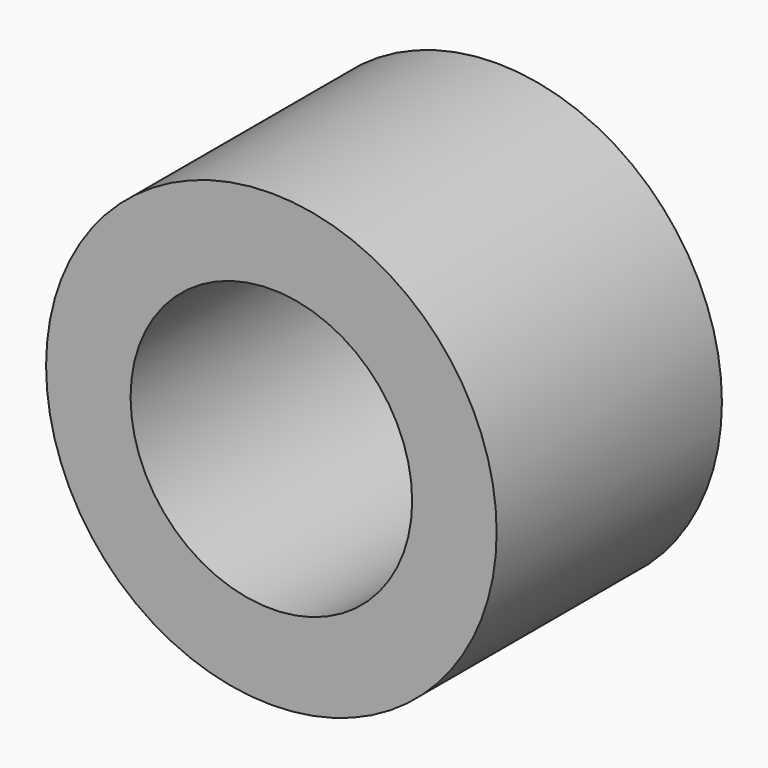
from build123d import *

# Parameters (mm, degrees)
F0_R     = 2.54
F0_R_2   = 1.5875
F1_DEPTH = 3.175


# Not quite as in the source:
# - a length typed as a fraction of an inch, garbled in the dataset ("3 / 203.2 mm" for 3/8 in), is restored


with BuildPart() as f1:
    # F0 (on Front) → F1 (new body)
    with BuildSketch(Plane.XZ):
        Circle(F0_R)
        Circle(F0_R_2, mode=Mode.SUBTRACT)
    extrude(amount=F1_DEPTH)


solid = f1.part
